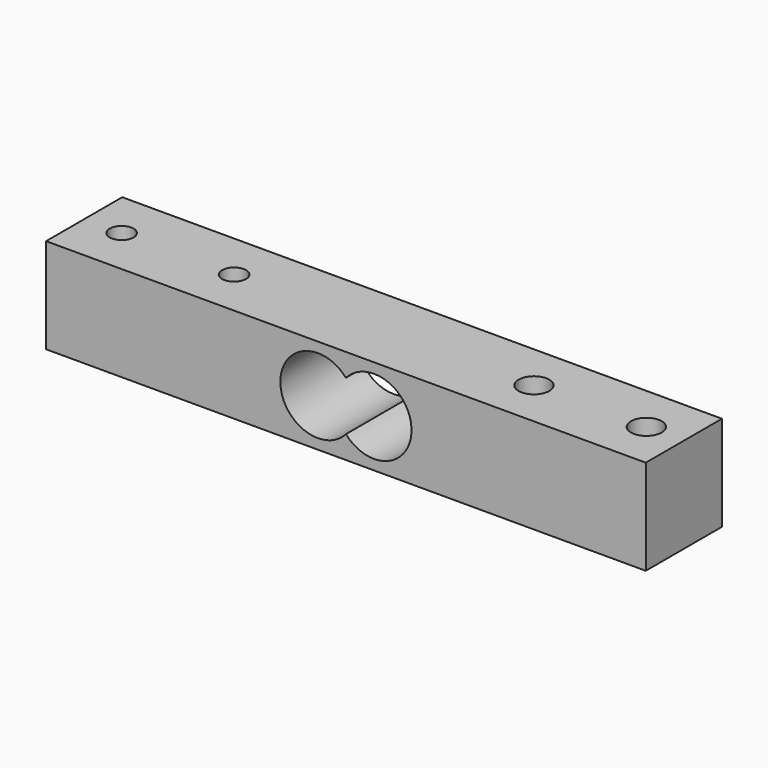
from build123d import *

# Parameters (mm, degrees)
F0_W     = 80
F0_H     = 12.7
F1_DEPTH = 12.7
F3_D     = 3.2
F5_D     = 4.1
F7_D     = 10


with BuildPart() as f1:
    # F0 (on Top) → F1 (new body)
    with BuildSketch(Plane.XY):
        Rectangle(F0_W, F0_H)
    extrude(amount=F1_DEPTH)

    # F3 (through all)
    with Locations(Plane.XY.offset(12.7)):
        with Locations((-35, 0), (-20, 0)):
            Hole(F3_D / 2)

    # F5 (through all)
    with Locations(Plane.XY.offset(12.7)):
        with Locations((20, 0), (35, 0)):
            Hole(F5_D / 2)

    # F7 (through all)
    with Locations(Plane.XZ.offset(6.35)):
        with Locations((-3.75, 6.35), (3.75, 6.35)):
            Hole(F7_D / 2)


solid = f1.part
